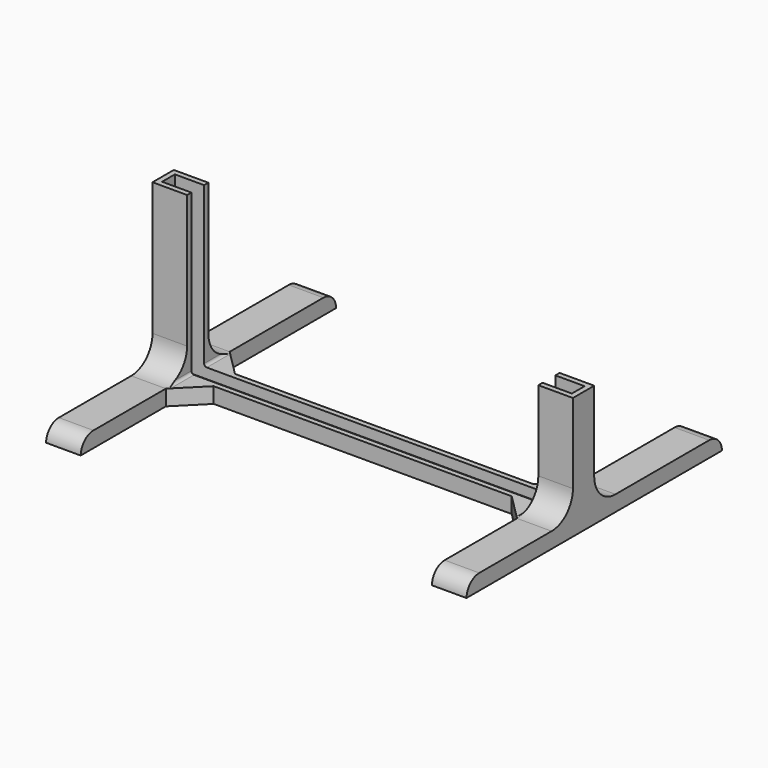
from build123d import *

# Parameters (mm, degrees)
F0_W         = 200.66
F0_H         = 3.7321411073
F1_DEPTH     = 12.7
F2_T         = -2.54
F3_W         = 16.51
F3_H         = 7.4579973676
F4_DEPTH     = 76.2
F6_START     = 11.176
F5_W         = 16.51
F5_H         = 7.4579973676
F6_DEPTH     = 65.024
F7_T1_DEPTH  = 7.4579973676
F8_T1_DEPTH  = 16.51
F8_T3_DEPTH  = 16.51
F9_T1_DEPTH  = 2.54
F9_T3_DEPTH  = 2.54
F9_T8_DEPTH  = 22.225
F9_S9_R      = 12.6999999999
F9_T10_DEPTH = 13
F9_T15_DEPTH = 22.225
F9_S16_R     = 12.6999999999
F9_T17_DEPTH = 13
F9_T22_DEPTH = 22.225
F9_S24_R     = 12.6999999999
F9_T25_DEPTH = 13
F9_T29_DEPTH = 22.225
F9_S31_R     = 12.6999999999
F9_T32_DEPTH = 13
F10_T1_DEPTH = 54.6013885108
F10_T3_DEPTH = 54.6013885108


# Not quite as in the source:
# - a fillet or chamfer that OpenCascade refuses, or shapes differently, is made with other operations: its cross-section is extruded or revolved along the edge and cut away or added


with BuildPart() as f1:
    # F0 (on Front) → F1 (new body)
    with BuildSketch(Plane.XZ):
        Polygon((83.82, -55.5934350035), (-83.82, -55.5934350035), (-83.82, 20.6065649965), (-100.33, 20.6065649965), (-100.33, -59.3192912638), (100.33, -59.3192912638), (100.33, -4.7934350035), (83.82, -4.7934350035), align=None)
        with Locations((0, -61.1853618175)):
            Rectangle(F0_W, F0_H)
    extrude(amount=F1_DEPTH)

    # F2
    f2_openings = [f1.faces().sort_by_distance(p)[0] for p in [
        (-92.075, -6.35, 20.606565),
        (-83.82, -6.35, -17.493435),
        (0, -6.35, -55.593435),
        (92.075, -6.35, -4.793435),
        (83.82, -6.35, -30.193435),
    ]]
    offset(amount=F2_T, openings=f2_openings)

    # F3 (on Front) → F4 (join)
    with BuildSketch(Plane.XZ):
        with Locations((92.075, -59.3224336873)):
            Rectangle(F3_W, F3_H)
        with Locations((-92.075, -59.3224336873)):
            Rectangle(F3_W, F3_H)
    extrude(amount=-F4_DEPTH)

    # F5 (on Front) → F6 (join)
    with BuildSketch(Plane.XZ.offset(F6_START)):
        with Locations((-92.075, -59.3224336873)):
            Rectangle(F5_W, F5_H)
        with Locations((92.075, -59.3224336873)):
            Rectangle(F5_W, F5_H)
    extrude(amount=F6_DEPTH)

    # F7: chamfer of 12.7 on 4 edges, made by hand

    # F7_s2 → F7_t1 (join)
    with BuildSketch(Plane.XY.offset(-63.0514323711)):
        Polygon((-71.12, -12.7), (-83.82, -25.4), (-83.82, -12.7), align=None)
        Polygon((-83.82, 12.7), (-71.12, 0), (-83.82, 0), align=None)
        Polygon((71.12, 0), (83.82, 12.7), (83.82, 0), align=None)
        Polygon((71.12, -12.7), (83.82, -25.4), (83.82, -12.7), align=None)
    extrude(amount=F7_T1_DEPTH)

    # F8: fillet of radius 12.7 on 4 edges, made by hand

    # F8_s2 → F8_t1 (join)
    with BuildSketch(Plane.YZ.offset(-100.33)):
        with BuildLine():
            ThreePointArc((-12.7, -42.8934350035), (-16.4197438789, -51.8736911246), (-25.4, -55.5934350035))
            Line((-25.4, -55.5934350035), (-12.7, -55.5934350035))
            Line((-12.7, -55.5934350035), (-12.7, -42.8934350035))
        make_face()
        with BuildLine():
            ThreePointArc((0, -42.8934350035), (3.7197438789, -51.8736911246), (12.7, -55.5934350035))
            Line((12.7, -55.5934350035), (0, -55.5934350035))
            Line((0, -55.5934350035), (0, -42.8934350035))
        make_face()
    extrude(amount=F8_T1_DEPTH)

    # F8_s4 → F8_t3 (join)
    with BuildSketch(Plane.YZ.offset(83.82)):
        with BuildLine():
            ThreePointArc((-25.4, -55.5934350035), (-16.4197438789, -51.8736911246), (-12.7, -42.8934350035))
            Line((-12.7, -42.8934350035), (-12.7, -55.5934350035))
            Line((-12.7, -55.5934350035), (-25.4, -55.5934350035))
        make_face()
        with BuildLine():
            ThreePointArc((12.7, -55.5934350035), (3.7197438789, -51.8736911246), (0, -42.8934350035))
            Line((0, -42.8934350035), (0, -55.5934350035))
            Line((0, -55.5934350035), (12.7, -55.5934350035))
        make_face()
    extrude(amount=F8_T3_DEPTH)

    # F9: fillet of radius 1.27 on 8 edges, made by hand

    # F9_s2 → F9_t1 (join)
    with BuildSketch(Plane.XZ):
        with BuildLine():
            ThreePointArc((-83.82, -54.3234350035), (-83.4480256121, -55.2214606156), (-82.55, -55.5934350035))
            Line((-82.55, -55.5934350035), (-83.82, -55.5934350035))
            Line((-83.82, -55.5934350035), (-83.82, -54.3234350035))
        make_face()
        with BuildLine():
            ThreePointArc((82.55, -55.5934350035), (83.4480256121, -55.2214606156), (83.82, -54.3234350035))
            Line((83.82, -54.3234350035), (83.82, -55.5934350035))
            Line((83.82, -55.5934350035), (82.55, -55.5934350035))
        make_face()
    extrude(amount=F9_T1_DEPTH)

    # F9_s4 → F9_t3 (join)
    with BuildSketch(Plane.XZ.offset(10.16)):
        with BuildLine():
            ThreePointArc((-83.82, -54.3234350035), (-83.4480256121, -55.2214606156), (-82.55, -55.5934350035))
            Line((-82.55, -55.5934350035), (-83.82, -55.5934350035))
            Line((-83.82, -55.5934350035), (-83.82, -54.3234350035))
        make_face()
        with BuildLine():
            ThreePointArc((82.55, -55.5934350035), (83.4480256121, -55.2214606156), (83.82, -54.3234350035))
            Line((83.82, -54.3234350035), (83.82, -55.5934350035))
            Line((83.82, -55.5934350035), (82.55, -55.5934350035))
        make_face()
    extrude(amount=F9_T3_DEPTH)


with BuildPart() as f9_tool6:
    # F9_s7 → F9_t8 (new body)
    with BuildSketch(Plane.XZ.offset(-22.225)):
        with BuildLine():
            ThreePointArc((-83.82, -54.3234350035), (-83.4480256121, -55.2214606156), (-82.55, -55.5934350035))
            Line((-82.55, -55.5934350035), (-83.82, -55.5934350035))
            Line((-83.82, -55.5934350035), (-83.82, -54.3234350035))
        make_face()
    extrude(amount=F9_T8_DEPTH)

    # F9_s9 → F9_t10 (cut, symmetric)
    with BuildSketch(Plane.YZ.offset(-83.2)):
        with Locations((12.6999999999, -42.8934350036)):
            Circle(F9_S9_R)
    extrude(amount=F9_T10_DEPTH, both=True, mode=Mode.SUBTRACT)

    split(bisect_by=Plane(origin=(-35.56, -35.56, 0), x_dir=(0, 0, 1), z_dir=(-0.7071067812, -0.7071067812, 0)), keep=Keep.TOP)


with BuildPart() as f1_1:
    add(f1.part)

    # F9_t5: union F9_tool6
    add(f9_tool6.part)


with BuildPart() as f9_tool13:
    # F9_s14 → F9_t15 (new body)
    with BuildSketch(Plane.XZ.offset(34.925)):
        with BuildLine():
            ThreePointArc((-83.82, -54.3234350035), (-83.4480256121, -55.2214606156), (-82.55, -55.5934350035))
            Line((-82.55, -55.5934350035), (-83.82, -55.5934350035))
            Line((-83.82, -55.5934350035), (-83.82, -54.3234350035))
        make_face()
    extrude(amount=-F9_T15_DEPTH)

    # F9_s16 → F9_t17 (cut, symmetric)
    with BuildSketch(Plane.YZ.offset(-83.2)):
        with Locations((-25.3999999999, -42.8934350036)):
            Circle(F9_S16_R)
    extrude(amount=F9_T17_DEPTH, both=True, mode=Mode.SUBTRACT)

    split(bisect_by=Plane(origin=(-29.21, 29.21, 0), x_dir=(0, 0, 1), z_dir=(-0.7071067812, 0.7071067812, 0)), keep=Keep.TOP)


with BuildPart() as f1_2:
    add(f1_1.part)

    # F9_t12: union F9_tool13
    add(f9_tool13.part)


with BuildPart() as f9_tool20:
    # F9_s21 → F9_t22 (new body)
    with BuildSketch(Plane.XZ):
        with BuildLine():
            ThreePointArc((82.55, -55.5934350035), (83.4480256121, -55.2214606156), (83.82, -54.3234350035))
            Line((83.82, -54.3234350035), (83.82, -55.5934350035))
            Line((83.82, -55.5934350035), (82.55, -55.5934350035))
        make_face()
    extrude(amount=-F9_T22_DEPTH)

    split(bisect_by=Plane(origin=(35.56, -35.56, 0), x_dir=(0, 0, 1), z_dir=(0.7071067812, -0.7071067812, 0)), keep=Keep.TOP)

    # F9_s24 → F9_t25 (cut, symmetric)
    with BuildSketch(Plane.YZ.offset(83.2)):
        with Locations((12.6999999999, -42.8934350036)):
            Circle(F9_S24_R)
    extrude(amount=F9_T25_DEPTH, both=True, mode=Mode.SUBTRACT)


with BuildPart() as f1_3:
    add(f1_2.part)

    # F9_t19: union F9_tool20
    add(f9_tool20.part)


with BuildPart() as f9_tool27:
    # F9_s28 → F9_t29 (new body)
    with BuildSketch(Plane.XZ.offset(12.7)):
        with BuildLine():
            ThreePointArc((82.55, -55.5934350035), (83.4480256121, -55.2214606156), (83.82, -54.3234350035))
            Line((83.82, -54.3234350035), (83.82, -55.5934350035))
            Line((83.82, -55.5934350035), (82.55, -55.5934350035))
        make_face()
    extrude(amount=F9_T29_DEPTH)

    split(bisect_by=Plane(origin=(29.21, 29.21, 0), x_dir=(0, 0, 1), z_dir=(0.7071067812, 0.7071067812, 0)), keep=Keep.TOP)

    # F9_s31 → F9_t32 (cut, symmetric)
    with BuildSketch(Plane.YZ.offset(83.2)):
        with Locations((-25.3999999999, -42.8934350036)):
            Circle(F9_S31_R)
    extrude(amount=F9_T32_DEPTH, both=True, mode=Mode.SUBTRACT)


with BuildPart() as f1_4:
    add(f1_3.part)

    # F9_t26: union F9_tool27
    add(f9_tool27.part)

    # F10: fillet of radius 7.62 on 4 edges, made by hand

    # F10_s2 → F10_t1 (cut)
    with BuildSketch(Plane.YZ.offset(-119.3756942554)):
        with BuildLine():
            ThreePointArc((68.5817222978, -55.5934350035), (73.9122916831, -57.7683059849), (76.2, -63.0514323711))
            Line((76.2, -63.0514323711), (76.2, -55.5934350035))
            Line((76.2, -55.5934350035), (68.5817222978, -55.5934350035))
        make_face()
        with BuildLine():
            ThreePointArc((-76.2, -63.0514323711), (-73.9122916831, -57.7683059849), (-68.5817222978, -55.5934350035))
            Line((-68.5817222978, -55.5934350035), (-76.2, -55.5934350035))
            Line((-76.2, -55.5934350035), (-76.2, -63.0514323711))
        make_face()
    extrude(amount=F10_T1_DEPTH, mode=Mode.SUBTRACT)

    # F10_s4 → F10_t3 (cut)
    with BuildSketch(Plane.YZ.offset(64.7743057446)):
        with BuildLine():
            ThreePointArc((68.5817222978, -55.5934350035), (73.9122916831, -57.7683059849), (76.2, -63.0514323711))
            Line((76.2, -63.0514323711), (76.2, -55.5934350035))
            Line((76.2, -55.5934350035), (68.5817222978, -55.5934350035))
        make_face()
        with BuildLine():
            ThreePointArc((-68.5817222978, -55.5934350035), (-73.9122916831, -57.7683059849), (-76.2, -63.0514323711))
            Line((-76.2, -63.0514323711), (-76.2, -55.5934350035))
            Line((-76.2, -55.5934350035), (-68.5817222978, -55.5934350035))
        make_face()
    extrude(amount=F10_T3_DEPTH, mode=Mode.SUBTRACT)


solid = f1_4.part
